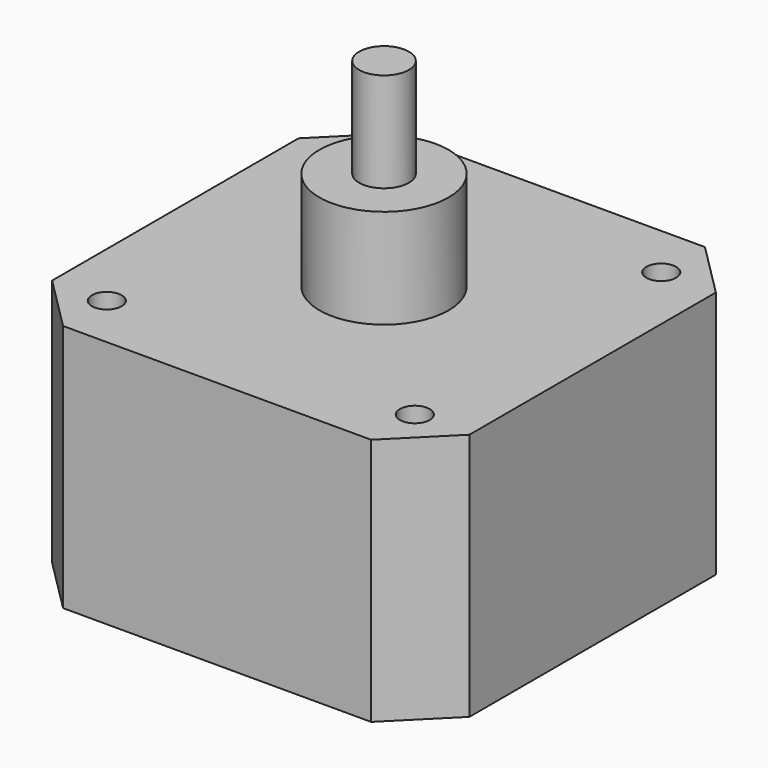
from build123d import *

# Parameters (mm, degrees)
F0_R     = 1.5
F0_R_2   = 6.5
F1_DEPTH = 25
F0_R_3   = 2.5
F2_DEPTH = 35
F3_DEPTH = 45


# Not quite as in the source:
# - a feature names something its author has since deleted; it is built from what else it names


with BuildPart() as f1:
    # F0 (on Top) → F1 (new body)
    with BuildSketch(Plane.XY):
        Polygon((15.5, 21), (-15.5, 21), (-21, 15.5), (-21, -15.5), (-15.5, -21), (15.5, -21), (21, -15.5), (21, 15.5), align=None)
        with Locations((-15.5, -15.5)):
            Circle(F0_R, mode=Mode.SUBTRACT)
        with Locations((15.5, -15.5)):
            Circle(F0_R, mode=Mode.SUBTRACT)
        with Locations((-15.5, 15.5)):
            Circle(F0_R, mode=Mode.SUBTRACT)
        Circle(F0_R_2, mode=Mode.SUBTRACT)
        with Locations((15.5, 15.5)):
            Circle(F0_R, mode=Mode.SUBTRACT)
    extrude(amount=F1_DEPTH)

    # F0 (on Top) → F2 (join)
    with BuildSketch(Plane.XY):
        Circle(F0_R_2)
        Circle(F0_R_3, mode=Mode.SUBTRACT)
    extrude(amount=F2_DEPTH)

    # F0 (on Top) → F3 (join)
    with BuildSketch(Plane.XY):
        Circle(F0_R_3)
    extrude(amount=F3_DEPTH)


solid = f1.part
